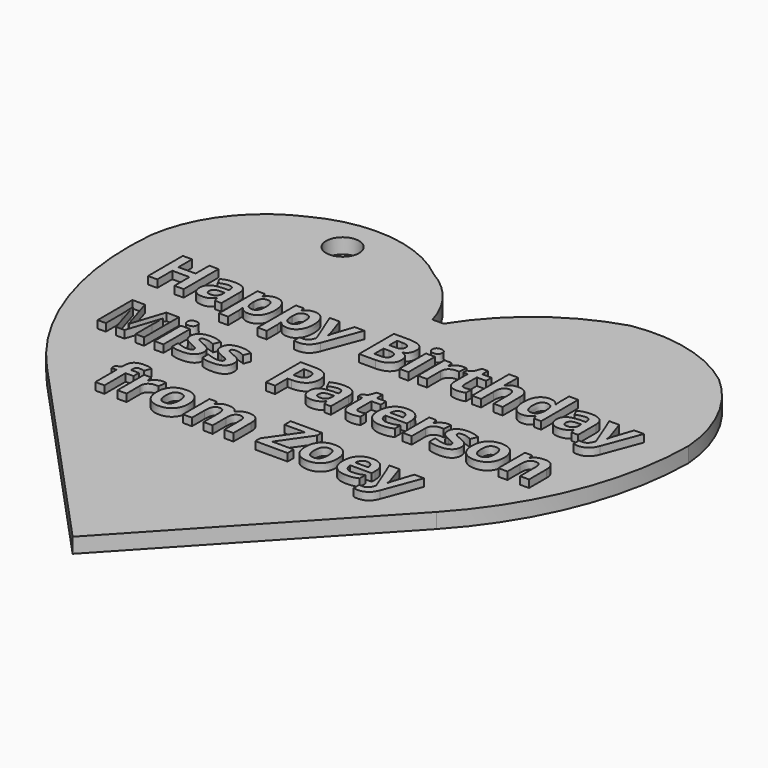
from build123d import *

# Parameters (mm, degrees)
F0_R         = 4.3853976727
F1_DEPTH     = 4
F2_TEXT_SIZE = 16.1648303568
F3_DEPTH     = 2


# Not quite as in the source:
# - Text() gives the source's letters only with a copy of the font that has no kerning and outlines rounded to 1/6400 em; it was checked with that copy


with BuildPart() as f1:
    # F0 (on Top) → F1 (new body)
    with BuildSketch(Plane.XY):
        with BuildLine():
            Line((-48.9956966412, -22.2974440235), (2.6404856421, -78.3344378687))
            Line((2.6404856421, -78.3344378687), (54.5590973669, -22.5590153551))
            ThreePointArc((54.5590973669, -22.5590153551), (70.9106831461, 3.2316430076), (76.8565413904, 33.1845925454))
            ThreePointArc((76.8565413904, 33.1845925454), (72.6310206768, 48.1759994182), (63.0673307689, 60.469621369))
            ThreePointArc((63.0673307689, 60.469621369), (49.1607224986, 67.188008855), (33.7285916997, 67.8043066759))
            ThreePointArc((33.7285916997, 67.8043066759), (16.2026802829, 58.8418542788), (2.9338740148, 44.3014999441))
            Line((2.9338740148, 44.3014999441), (0, 44.3014999441))
            ThreePointArc((0, 44.3014999441), (-4.7137449351, 53.6159378813), (-12.615659289, 60.4378067559))
            ThreePointArc((-12.615659289, 60.4378067559), (-30.2285086, 67.8501321318), (-48.9956966412, 64.2518434608))
            ThreePointArc((-48.9956966412, 64.2518434608), (-62.571777714, 53.521847615), (-69.2394282608, 37.5535908431))
            ThreePointArc((-69.2394282608, 37.5535908431), (-65.4708296565, 5.4791742888), (-48.9956966412, -22.2974440235))
        make_face()
        with Locations((-34.8838306963, 58.1092759967)):
            Circle(F0_R, mode=Mode.SUBTRACT)
    extrude(amount=F1_DEPTH)

    # F2 (on face) → F3 (join)
    with BuildSketch(Plane.XY.offset(4)):
        with Locations((-57.2937152997, 19.7833457915)):
            Text('Happy Birthday', F2_TEXT_SIZE, font='Open Sans', font_style=FontStyle.BOLD, text_align=(TextAlign.LEFT, TextAlign.BOTTOM))
        with Locations((-53.0933851616, -2.2008234938)):
            Text('Miss  Paterson', F2_TEXT_SIZE, font='Open Sans', font_style=FontStyle.BOLD, text_align=(TextAlign.LEFT, TextAlign.BOTTOM))
        with Locations((-36.2920646096, -24.184992779)):
            Text('from Zoey', F2_TEXT_SIZE, font='Open Sans', font_style=FontStyle.BOLD, text_align=(TextAlign.LEFT, TextAlign.BOTTOM))
    extrude(amount=F3_DEPTH)


solid = f1.part
